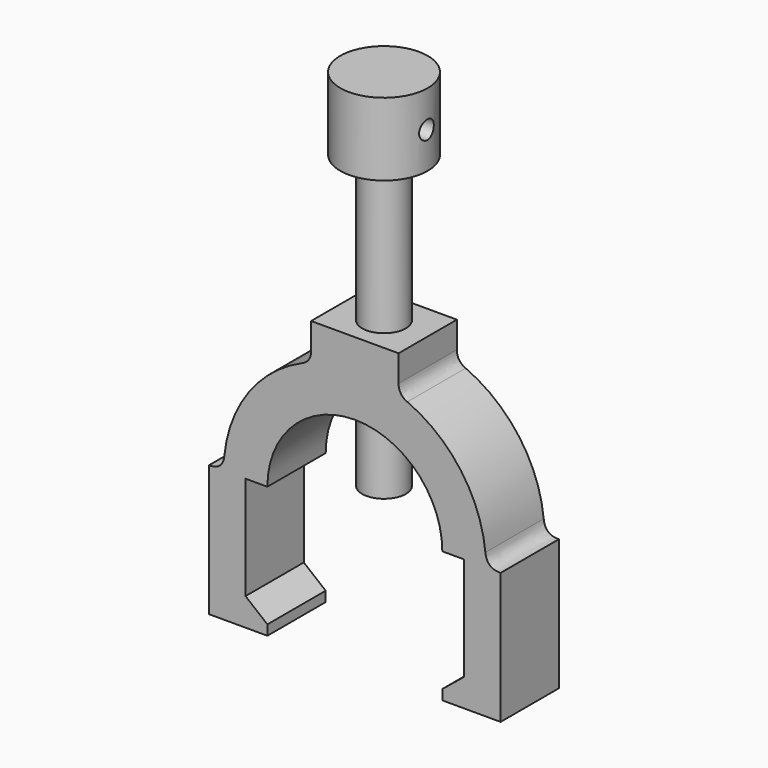
from build123d import *

# Parameters (mm, degrees)
F1_DEPTH      = 20
F2_R          = 6
F3_DEPTH      = 40
F3_DEPTH_BACK = 40
F4_R          = 12
F5_DEPTH      = 20
F7_R          = 2.5
F8_DEPTH      = 25
F9_T1_DEPTH   = 20


# Not quite as in the source:
# - a fillet or chamfer that OpenCascade refuses, or shapes differently, is made with other operations: its cross-section is extruded or revolved along the edge and cut away or added
# - a feature names something its author has since deleted; it is built from what else it names


with BuildPart() as f1:
    # F0 (on Front) → F1 (new body)
    with BuildSketch(Plane.XZ):
        with BuildLine():
            ThreePointArc((-12, 33.941125497), (-29.3938769134, 20.7846096908), (-36, 0))
            Line((-36, 0), (-30, 0))
            Line((-30, 0), (-24, 0))
            ThreePointArc((-24, 0), (0, 24), (24, 0))
            Line((24, 0), (30, 0))
            Line((30, 0), (36, 0))
            ThreePointArc((36, 0), (29.3938769134, 20.7846096908), (12, 33.941125497))
            Line((12, 33.941125497), (12, 43.941125497))
            Line((12, 43.941125497), (-12, 43.941125497))
            Line((-12, 43.941125497), (-12, 33.941125497))
        make_face()
        Polygon((-30, 0), (-36, 0), (-40, 0), (-40, -28.374), (-40, -36), (-24, -36), (-24, -33.2482792437), (-30, -28.374), align=None)
        Polygon((36, 0), (30, 0), (30, -28.374), (24, -33.2482792437), (24, -36), (40, -36), (40, -28.374), (40, 0), align=None)
    extrude(amount=F1_DEPTH)

    # F2 (on face) → F3 (join, two sides)
    with BuildSketch(Plane.XY.offset(43.941125497)) as f3_sk:
        with Locations((0, -10)):
            Circle(F2_R)
    extrude(amount=F3_DEPTH)
    extrude(f3_sk.sketch, amount=-F3_DEPTH_BACK)

    # F4 (on face) → F5 (join)
    with BuildSketch(Plane.XY.offset(83.941125497)):
        with Locations((0, -10)):
            Circle(F4_R)
    extrude(amount=F5_DEPTH)

    # F7 (on offset) → F8 (cut)
    with BuildSketch(Plane.YZ.offset(12)):
        with Locations((-10.1158004254, 93.941125497)):
            Circle(F7_R)
    extrude(amount=-F8_DEPTH, mode=Mode.SUBTRACT)

    # F9: fillet of radius 4 on 4 edges, made by hand

    # F9_s2 → F9_t1 (join)
    with BuildSketch(Plane.XZ):
        with BuildLine():
            add(Edge.make_bspline(
                [(35.8195477358, 3.6), (36.1813613493, 0), (39.7994974843, 0)],
                knots=[0, 0, 0, 1, 1, 1], degree=2, weights=[1, 1, 1]))
            Line((39.7994974843, 0), (36, 0))
            ThreePointArc((36, 0), (35.954858632, 1.8022599022), (35.8195477358, 3.6))
        make_face()
        with BuildLine():
            add(Edge.make_bspline(
                [(-35.8195477358, 3.6), (-36.1813613493, 0), (-39.7994974843, 0)],
                knots=[0, 0, 0, 1, 1, 1], degree=2, weights=[1, 1, 1]))
            Line((-39.7994974843, 0), (-36, 0))
            ThreePointArc((-36, 0), (-35.954858632, 1.8022599022), (-35.8195477358, 3.6))
        make_face()
        with BuildLine():
            add(Edge.make_bspline(
                [(-12, 36.6606055596), (-12, 34.0419908768), (-14.4, 32.9945450037)],
                knots=[0, 0, 0, 1, 1, 1], degree=2, weights=[1, 1, 1]))
            ThreePointArc((-14.4, 32.9945450037), (-13.2084822617, 33.4893415334), (-12, 33.941125497))
            Line((-12, 33.941125497), (-12, 36.6606055596))
        make_face()
        with BuildLine():
            add(Edge.make_bspline(
                [(12, 36.6606055596), (12, 34.0419908768), (14.4, 32.9945450037)],
                knots=[0, 0, 0, 1, 1, 1], degree=2, weights=[1, 1, 1]))
            ThreePointArc((14.4, 32.9945450037), (13.2084822617, 33.4893415334), (12, 33.941125497))
            Line((12, 33.941125497), (12, 36.6606055596))
        make_face()
    extrude(amount=F9_T1_DEPTH)


solid = f1.part
